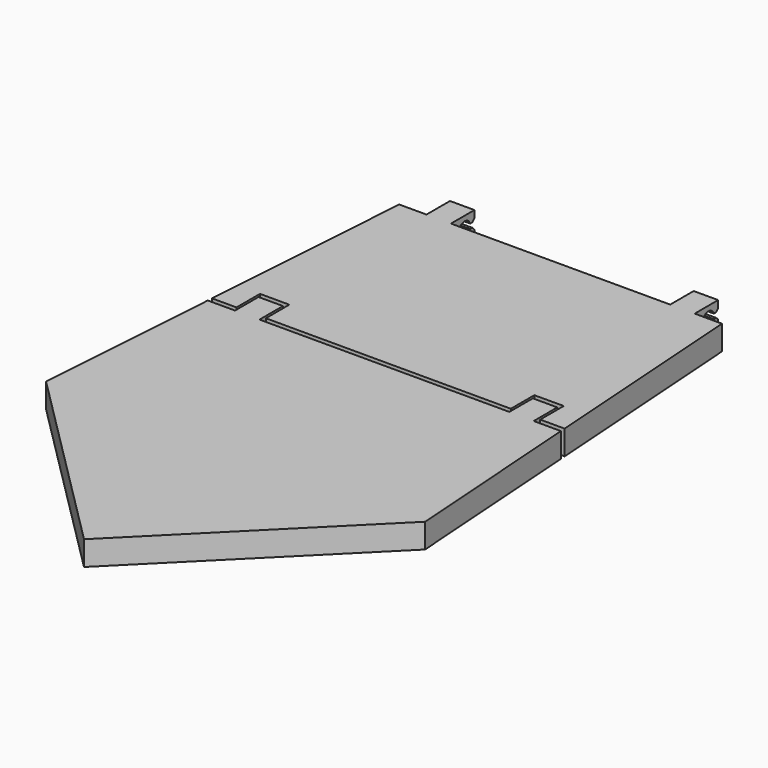
from build123d import *

# Parameters (mm, degrees)
F1_DEPTH = 5
F4_DEPTH = 72.8
F5_SIZE  = 0.5
F8_START = -7
F7_R     = 1.5
F7_R_2   = 1
F8_DEPTH = 68.5
F9_START = -5.6
F9_DEPTH = 68.7


with BuildPart() as f1:
    # F0 (on Top) → F1 (new body)
    with BuildSketch(Plane.XY):
        Polygon((-36.1032915569, -18.1079245215), (-38.7457432998, -56.1079245215), (0.0188927832, -94.8725606045), (38.7457432998, -56.145710088), (36.10329, -18.1457101963), (30.53375, -18.1457101963), (30.53375, -12.1079245215), (25.53375, -12.1079245215), (25.53375, -17.1079245215), (25.53375, -18.1079245215), (-25.5337533532, -18.1079245215), (-25.5337533532, -12.1079245215), (-30.5337533532, -12.1079245215), (-30.5337533532, -18.1079245215), align=None)
    extrude(amount=F1_DEPTH)

    # F7 (on offset) → F8 (cut)
    with BuildSketch(Plane.YZ.offset(40.53375).offset(F8_START)):
        with Locations((-14.6457101963, 2.5)):
            Circle(F7_R)
        with Locations((-14.6457101963, 2.5)):
            Circle(F7_R_2, mode=Mode.SUBTRACT)
    extrude(amount=-F8_DEPTH, mode=Mode.SUBTRACT)



with BuildPart() as f1b:
    # F0 (on Top) → F1, piece 2 (new body)
    with BuildSketch(Plane.XY):
        Polygon((-36.0337533532, -17.1079245215), (-31.0337533532, -17.1079245215), (-31.0337533532, -11.1079245215), (-25.0337533532, -11.1079245215), (-25.0337533532, -17.1079245215), (25.03375, -17.1079245215), (25.03375, -11.1079245215), (31.03375, -11.0867864177), (31.03375, -17.1079245215), (36.03375, -17.1079245215), (32.974534184, 26.8920754785), (27.404534184, 26.8920754785), (27.404534184, 32.8920754785), (22.404534184, 32.8920754785), (22.404534184, 26.8920754785), (-22.404534184, 26.8920754785), (-22.404534184, 32.8920754785), (-27.404534184, 32.8920754785), (-27.404534184, 26.8920754785), (-32.9740723878, 26.8920754785), align=None)
    extrude(amount=F1_DEPTH)

    # F3 (on offset) → F4 (cut)
    with BuildSketch(Plane.YZ.offset(37.404534184)):
        with BuildLine():
            Line((34.7708482201, 3), (31.8062890408, 3))
            ThreePointArc((31.8062890408, 3), (30.2629438912, 3.9944313411), (28.9130555327, 2.75))
            Line((28.9130555327, 2.75), (27.8920754785, 2.75))
            Line((27.8920754785, 2.75), (27.8920754785, 2.25))
            Line((27.8920754785, 2.25), (28.9130555327, 2.25))
            ThreePointArc((28.9130555327, 2.25), (30.2629438912, 1.0055686589), (31.8062890408, 2))
            Line((31.8062890408, 2), (34.7708482201, 2))
            Line((34.7708482201, 2), (34.7708482201, 3))
        make_face()
    extrude(amount=-F4_DEPTH, mode=Mode.SUBTRACT)

    # F5
    f5_edges = [f1b.edges().sort_by_distance(p)[0] for p in [
        (24.904534, 32.892075, 3),
        (24.904534, 32.892075, 2),
        (-24.904534, 32.892075, 3),
        (-24.904534, 32.892075, 2),
    ]]
    chamfer(f5_edges, length=F5_SIZE)


with BuildPart() as f1_1:
    add(f1.part)

    add(f1b.part)  # F9 merges F1b
    # F7 (on offset) → F9 (join)
    with BuildSketch(Plane.YZ.offset(40.53375).offset(F9_START)):
        with Locations((-14.6457101963, 2.5)):
            Circle(F7_R_2)
    extrude(amount=-F9_DEPTH)


solid = f1_1.part
